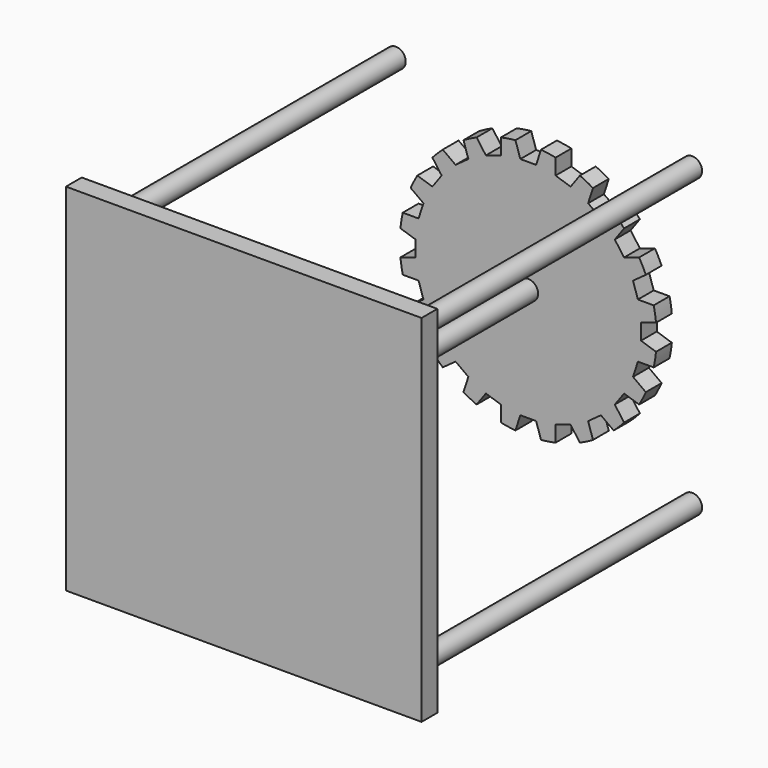
from build123d import *

# Parameters (mm, degrees)
F0_W      = 90
F0_H      = 90
F1_DEPTH  = 5
F2_R      = 2.5
F3_DEPTH  = 90
F4_R      = 2.5
F5_DEPTH  = 90
F6_R      = 32.5
F7_DEPTH  = 5
F10_DEPTH = 10
F11_COUNT = 20
F12_DEPTH = 25


with BuildPart() as f1:
    # F0 (on Front) → F1 (new body)
    with BuildSketch(Plane.XZ):
        Rectangle(F0_W, F0_H)
    extrude(amount=F1_DEPTH)

    # F2 (on face) → F3 (join)
    with BuildSketch(Plane(origin=(0, 0, 0), x_dir=(-1, 0, 0), z_dir=(0, 1, 0))):
        Circle(F2_R)
    extrude(amount=F3_DEPTH)

    # F4 (on face) → F5 (join)
    with BuildSketch(Plane(origin=(0, 0, 0), x_dir=(-1, 0, 0), z_dir=(0, 1, 0))):
        with Locations((-37.5, 37.5)):
            Circle(F4_R)
        with Locations((37.5, 37.5)):
            Circle(F4_R)
        with Locations((37.5, -37.5)):
            Circle(F4_R)
        with Locations((-37.5, -37.5)):
            Circle(F4_R)
    extrude(amount=F5_DEPTH)


with BuildPart() as f7:
    # F6 (on face) → F7 (new body)
    with BuildSketch(Plane(origin=(0, 90, 0), x_dir=(-1, 0, 0), z_dir=(0, 1, 0))):
        Circle(F6_R)
    extrude(amount=-F7_DEPTH)

    # F9 (on face) → F10 (join)
    with BuildSketch(Plane(origin=(0, 90, 0), x_dir=(-1, 0, 0), z_dir=(0, 1, 0))):
        with BuildLine():
            Line((2, 28.5342628303), (3.2360679775, 32.3384888955))
            ThreePointArc((3.2360679775, 32.3384888955), (0, 33.490093397), (-3.2360679775, 32.3384888955))
            Line((-3.2360679775, 32.3384888955), (-2, 28.5342628303))
            Line((-2, 28.5342628303), (2, 28.5342628303))
        make_face()
    extrude(amount=F10_DEPTH)


with BuildPart() as f11_1:
    # F11: instance of F7
    add(f7.part.rotate(Axis((0, 90, 0), (0, 1, 0)), 1 * 360 / F11_COUNT))


with BuildPart() as f11_2:
    # F11: instance of F7
    add(f7.part.rotate(Axis((0, 90, 0), (0, 1, 0)), 2 * 360 / F11_COUNT))


with BuildPart() as f11_3:
    # F11: instance of F7
    add(f7.part.rotate(Axis((0, 90, 0), (0, 1, 0)), 3 * 360 / F11_COUNT))


with BuildPart() as f11_4:
    # F11: instance of F7
    add(f7.part.rotate(Axis((0, 90, 0), (0, 1, 0)), 4 * 360 / F11_COUNT))


with BuildPart() as f11_5:
    # F11: instance of F7
    add(f7.part.rotate(Axis((0, 90, 0), (0, 1, 0)), 5 * 360 / F11_COUNT))


with BuildPart() as f11_6:
    # F11: instance of F7
    add(f7.part.rotate(Axis((0, 90, 0), (0, 1, 0)), 6 * 360 / F11_COUNT))


with BuildPart() as f11_7:
    # F11: instance of F7
    add(f7.part.rotate(Axis((0, 90, 0), (0, 1, 0)), 7 * 360 / F11_COUNT))


with BuildPart() as f11_8:
    # F11: instance of F7
    add(f7.part.rotate(Axis((0, 90, 0), (0, 1, 0)), 8 * 360 / F11_COUNT))


with BuildPart() as f11_9:
    # F11: instance of F7
    add(f7.part.rotate(Axis((0, 90, 0), (0, 1, 0)), 9 * 360 / F11_COUNT))


with BuildPart() as f11_10:
    # F11: instance of F7
    add(f7.part.rotate(Axis((0, 90, 0), (0, 1, 0)), 10 * 360 / F11_COUNT))


with BuildPart() as f11_11:
    # F11: instance of F7
    add(f7.part.rotate(Axis((0, 90, 0), (0, 1, 0)), 11 * 360 / F11_COUNT))


with BuildPart() as f11_12:
    # F11: instance of F7
    add(f7.part.rotate(Axis((0, 90, 0), (0, 1, 0)), 12 * 360 / F11_COUNT))


with BuildPart() as f11_13:
    # F11: instance of F7
    add(f7.part.rotate(Axis((0, 90, 0), (0, 1, 0)), 13 * 360 / F11_COUNT))


with BuildPart() as f11_14:
    # F11: instance of F7
    add(f7.part.rotate(Axis((0, 90, 0), (0, 1, 0)), 14 * 360 / F11_COUNT))


with BuildPart() as f11_15:
    # F11: instance of F7
    add(f7.part.rotate(Axis((0, 90, 0), (0, 1, 0)), 15 * 360 / F11_COUNT))


with BuildPart() as f11_16:
    # F11: instance of F7
    add(f7.part.rotate(Axis((0, 90, 0), (0, 1, 0)), 16 * 360 / F11_COUNT))


with BuildPart() as f11_17:
    # F11: instance of F7
    add(f7.part.rotate(Axis((0, 90, 0), (0, 1, 0)), 17 * 360 / F11_COUNT))


with BuildPart() as f11_18:
    # F11: instance of F7
    add(f7.part.rotate(Axis((0, 90, 0), (0, 1, 0)), 18 * 360 / F11_COUNT))


with BuildPart() as f11_19:
    # F11: instance of F7
    add(f7.part.rotate(Axis((0, 90, 0), (0, 1, 0)), 19 * 360 / F11_COUNT))


with BuildPart() as f12_tool:
    # F11_face (on face) + F10_face (on face) → F12 (new body)
    with BuildSketch(Plane(origin=(9.5911509304, 100, 29.5185273212), x_dir=(-1, 0, 0), z_dir=(0, 1, 0))):
        with BuildLine():
            Line((-3.4796752479, 0.23720327), (-1.1285342387, -2.9988647075))
            Line((-1.1285342387, -2.9988647075), (2.6756918265, -1.76279673))
            Line((2.6756918265, -1.76279673), (2.6756918265, 2.23720327))
            ThreePointArc((2.6756918265, 2.23720327), (-0.7578570724, 2.3324442354), (-3.4796752479, 0.23720327))
        make_face()
        with BuildLine():
            Line((-12.0349699125, -5.2582532649), (-8.798901935, -7.6093942741))
            Line((-8.798901935, -7.6093942741), (-5.5628339575, -5.2582532649))
            Line((-5.5628339575, -5.2582532649), (-6.798901935, -1.4540271997))
            ThreePointArc((-6.798901935, -1.4540271997), (-10.0938320662, -2.4244726198), (-12.0349699125, -5.2582532649))
        make_face()
        with BuildLine():
            Line((16.5066100344, 2.23720327), (16.5066100344, -1.76279673))
            Line((16.5066100344, -1.76279673), (20.3108360996, -2.9988647075))
            Line((20.3108360996, -2.9988647075), (22.6619771087, 0.23720327))
            ThreePointArc((22.6619771087, 0.23720327), (19.9401589333, 2.3324442354), (16.5066100344, 2.23720327))
        make_face()
        with BuildLine():
            Line((25.9812037959, -1.4540271997), (24.7451358184, -5.2582532649))
            Line((24.7451358184, -5.2582532649), (27.9812037959, -7.6093942741))
            Line((27.9812037959, -7.6093942741), (31.2172717734, -5.2582532649))
            ThreePointArc((31.2172717734, -5.2582532649), (29.2761339271, -2.4244726198), (25.9812037959, -1.4540271997))
        make_face()
        with BuildLine():
            Line((33.8514249867, -7.8924064782), (31.5002839776, -11.1284744557))
            Line((31.5002839776, -11.1284744557), (33.8514249867, -14.3645424332))
            Line((33.8514249867, -14.3645424332), (37.6556510519, -13.1284744557))
            ThreePointArc((37.6556510519, -13.1284744557), (36.6852056318, -9.8335443245), (33.8514249867, -7.8924064782))
        make_face()
        with BuildLine():
            Line((39.3468815217, -16.4477011429), (36.1108135442, -18.798842152))
            Line((36.1108135442, -18.798842152), (37.3468815217, -22.6030682172))
            Line((37.3468815217, -22.6030682172), (41.3468815217, -22.6030682172))
            ThreePointArc((41.3468815217, -22.6030682172), (41.442122487, -19.1695193183), (39.3468815217, -16.4477011429))
        make_face()
        with BuildLine():
            Line((41.9296398259, -26.2824593437), (38.1254137608, -27.5185273212))
            Line((38.1254137608, -27.5185273212), (38.1254137608, -31.5185273212))
            Line((38.1254137608, -31.5185273212), (41.9296398259, -32.7545952987))
            ThreePointArc((41.9296398259, -32.7545952987), (43.0812443274, -29.5185273212), (41.9296398259, -26.2824593437))
        make_face()
        with BuildLine():
            Line((41.3468815217, -36.4339864251), (37.3468815217, -36.4339864251))
            Line((37.3468815217, -36.4339864251), (36.1108135442, -40.2382124903))
            Line((36.1108135442, -40.2382124903), (39.3468815217, -42.5893534995))
            ThreePointArc((39.3468815217, -42.5893534995), (41.442122487, -39.867535324), (41.3468815217, -36.4339864251))
        make_face()
        with BuildLine():
            Line((-18.473349191, -13.1284744557), (-14.6691231258, -14.3645424332))
            Line((-14.6691231258, -14.3645424332), (-12.3179821167, -11.1284744557))
            Line((-12.3179821167, -11.1284744557), (-14.6691231258, -7.8924064782))
            ThreePointArc((-14.6691231258, -7.8924064782), (-17.5029037709, -9.8335443245), (-18.473349191, -13.1284744557))
        make_face()
        with BuildLine():
            Line((-22.1645796608, -22.6030682172), (-18.1645796608, -22.6030682172))
            Line((-18.1645796608, -22.6030682172), (-16.9285116833, -18.798842152))
            Line((-16.9285116833, -18.798842152), (-20.1645796608, -16.4477011429))
            ThreePointArc((-20.1645796608, -16.4477011429), (-22.2598206261, -19.1695193183), (-22.1645796608, -22.6030682172))
        make_face()
        with BuildLine():
            Line((-22.7473379651, -32.7545952987), (-18.9431118999, -31.5185273212))
            Line((-18.9431118999, -31.5185273212), (-18.9431118999, -27.5185273212))
            Line((-18.9431118999, -27.5185273212), (-22.7473379651, -26.2824593437))
            ThreePointArc((-22.7473379651, -26.2824593437), (-23.8989424665, -29.5185273212), (-22.7473379651, -32.7545952987))
        make_face()
        with BuildLine():
            Line((-20.1645796608, -42.5893534995), (-16.9285116833, -40.2382124903))
            Line((-16.9285116833, -40.2382124903), (-18.1645796608, -36.4339864251))
            Line((-18.1645796608, -36.4339864251), (-22.1645796608, -36.4339864251))
            ThreePointArc((-22.1645796608, -36.4339864251), (-22.2598206261, -39.867535324), (-20.1645796608, -42.5893534995))
        make_face()
        with BuildLine():
            Line((-14.6691231258, -51.1446481641), (-12.3179821167, -47.9085801866))
            Line((-12.3179821167, -47.9085801866), (-14.6691231258, -44.6725122091))
            Line((-14.6691231258, -44.6725122091), (-18.473349191, -45.9085801866))
            ThreePointArc((-18.473349191, -45.9085801866), (-17.5029037709, -49.2035103178), (-14.6691231258, -51.1446481641))
        make_face()
        with BuildLine():
            Line((-6.798901935, -57.5830274426), (-5.5628339575, -53.7788013775))
            Line((-5.5628339575, -53.7788013775), (-8.798901935, -51.4276603683))
            Line((-8.798901935, -51.4276603683), (-12.0349699125, -53.7788013775))
            ThreePointArc((-12.0349699125, -53.7788013775), (-10.0938320662, -56.6125820225), (-6.798901935, -57.5830274426))
        make_face()
        with BuildLine():
            Line((2.6756918265, -61.2742579124), (2.6756918265, -57.2742579124))
            Line((2.6756918265, -57.2742579124), (-1.1285342387, -56.0381899349))
            Line((-1.1285342387, -56.0381899349), (-3.4796752479, -59.2742579124))
            ThreePointArc((-3.4796752479, -59.2742579124), (-0.7578570724, -61.3694988777), (2.6756918265, -61.2742579124))
        make_face()
        with BuildLine():
            Line((12.8272189079, -61.8570162167), (11.5911509304, -58.0527901515))
            Line((11.5911509304, -58.0527901515), (7.5911509304, -58.0527901515))
            Line((7.5911509304, -58.0527901515), (6.3550829529, -61.8570162167))
            ThreePointArc((6.3550829529, -61.8570162167), (9.5911509304, -63.0086207181), (12.8272189079, -61.8570162167))
        make_face()
        with BuildLine():
            Line((22.6619771087, -59.2742579124), (20.3108360996, -56.0381899349))
            Line((20.3108360996, -56.0381899349), (16.5066100344, -57.2742579124))
            Line((16.5066100344, -57.2742579124), (16.5066100344, -61.2742579124))
            ThreePointArc((16.5066100344, -61.2742579124), (19.9401589333, -61.3694988777), (22.6619771087, -59.2742579124))
        make_face()
        with BuildLine():
            Line((31.2172717734, -53.7788013775), (27.9812037959, -51.4276603683))
            Line((27.9812037959, -51.4276603683), (24.7451358184, -53.7788013775))
            Line((24.7451358184, -53.7788013775), (25.9812037959, -57.5830274426))
            ThreePointArc((25.9812037959, -57.5830274426), (29.2761339271, -56.6125820225), (31.2172717734, -53.7788013775))
        make_face()
        with BuildLine():
            Line((37.6556510519, -45.9085801866), (33.8514249867, -44.6725122091))
            Line((33.8514249867, -44.6725122091), (31.5002839776, -47.9085801866))
            Line((31.5002839776, -47.9085801866), (33.8514249867, -51.1446481641))
            ThreePointArc((33.8514249867, -51.1446481641), (36.6852056318, -49.2035103178), (37.6556510519, -45.9085801866))
        make_face()
    with BuildSketch(Plane(origin=(0, 100, 31.0376163934), x_dir=(-1, 0, 0), z_dir=(0, 1, 0))):
        with BuildLine():
            Line((-3.2360679775, 1.3008725022), (-2, -2.503353563))
            Line((-2, -2.503353563), (2, -2.503353563))
            Line((2, -2.503353563), (3.2360679775, 1.3008725022))
            ThreePointArc((3.2360679775, 1.3008725022), (0, 2.4524770036), (-3.2360679775, 1.3008725022))
        make_face()
    extrude(amount=-F12_DEPTH)


with BuildPart() as f7_1:
    add(f7.part)

    # F12: cut by f12_tool
    add(f12_tool.part, mode=Mode.SUBTRACT)


with BuildPart() as f11_1_1:
    add(f11_1.part)

    # F12: cut by f12_tool
    add(f12_tool.part, mode=Mode.SUBTRACT)


with BuildPart() as f11_2_1:
    add(f11_2.part)

    # F12: cut by f12_tool
    add(f12_tool.part, mode=Mode.SUBTRACT)


with BuildPart() as f11_3_1:
    add(f11_3.part)

    # F12: cut by f12_tool
    add(f12_tool.part, mode=Mode.SUBTRACT)


with BuildPart() as f11_4_1:
    add(f11_4.part)

    # F12: cut by f12_tool
    add(f12_tool.part, mode=Mode.SUBTRACT)


with BuildPart() as f11_5_1:
    add(f11_5.part)

    # F12: cut by f12_tool
    add(f12_tool.part, mode=Mode.SUBTRACT)


with BuildPart() as f11_6_1:
    add(f11_6.part)

    # F12: cut by f12_tool
    add(f12_tool.part, mode=Mode.SUBTRACT)


with BuildPart() as f11_7_1:
    add(f11_7.part)

    # F12: cut by f12_tool
    add(f12_tool.part, mode=Mode.SUBTRACT)


with BuildPart() as f11_8_1:
    add(f11_8.part)

    # F12: cut by f12_tool
    add(f12_tool.part, mode=Mode.SUBTRACT)


with BuildPart() as f11_9_1:
    add(f11_9.part)

    # F12: cut by f12_tool
    add(f12_tool.part, mode=Mode.SUBTRACT)


with BuildPart() as f11_10_1:
    add(f11_10.part)

    # F12: cut by f12_tool
    add(f12_tool.part, mode=Mode.SUBTRACT)


with BuildPart() as f11_11_1:
    add(f11_11.part)

    # F12: cut by f12_tool
    add(f12_tool.part, mode=Mode.SUBTRACT)


with BuildPart() as f11_12_1:
    add(f11_12.part)

    # F12: cut by f12_tool
    add(f12_tool.part, mode=Mode.SUBTRACT)


with BuildPart() as f11_13_1:
    add(f11_13.part)

    # F12: cut by f12_tool
    add(f12_tool.part, mode=Mode.SUBTRACT)


with BuildPart() as f11_14_1:
    add(f11_14.part)

    # F12: cut by f12_tool
    add(f12_tool.part, mode=Mode.SUBTRACT)


with BuildPart() as f11_15_1:
    add(f11_15.part)

    # F12: cut by f12_tool
    add(f12_tool.part, mode=Mode.SUBTRACT)


with BuildPart() as f11_16_1:
    add(f11_16.part)

    # F12: cut by f12_tool
    add(f12_tool.part, mode=Mode.SUBTRACT)


with BuildPart() as f11_17_1:
    add(f11_17.part)

    # F12: cut by f12_tool
    add(f12_tool.part, mode=Mode.SUBTRACT)


with BuildPart() as f11_18_1:
    add(f11_18.part)

    # F12: cut by f12_tool
    add(f12_tool.part, mode=Mode.SUBTRACT)


with BuildPart() as f11_19_1:
    add(f11_19.part)

    # F12: cut by f12_tool
    add(f12_tool.part, mode=Mode.SUBTRACT)


solid = Compound([f1.part, f7_1.part, f11_1_1.part, f11_2_1.part, f11_3_1.part, f11_4_1.part, f11_5_1.part, f11_6_1.part, f11_7_1.part, f11_8_1.part, f11_9_1.part, f11_10_1.part, f11_11_1.part, f11_12_1.part, f11_13_1.part, f11_14_1.part, f11_15_1.part, f11_16_1.part, f11_17_1.part, f11_18_1.part, f11_19_1.part])
